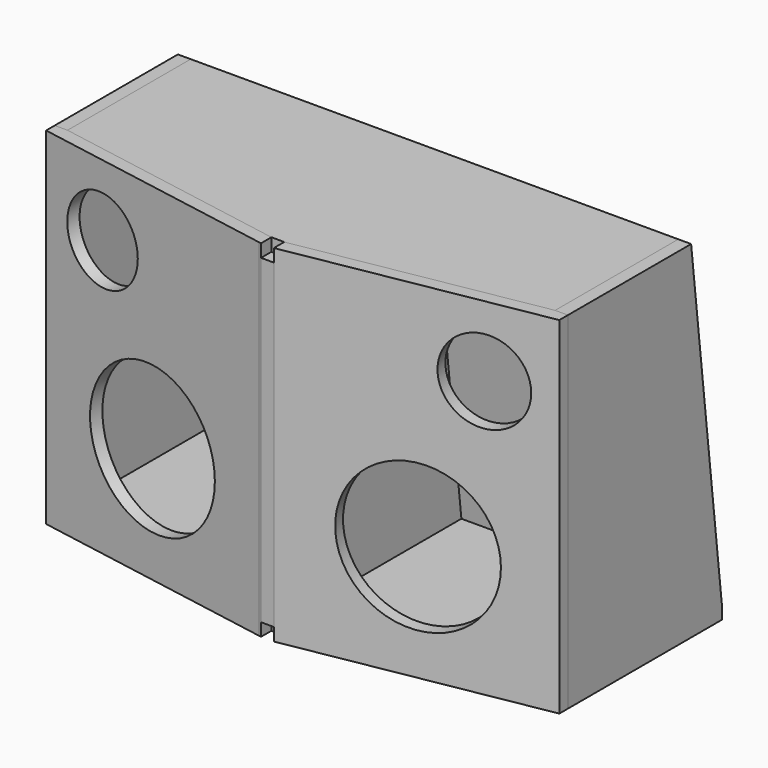
from build123d import *

# Parameters (mm, degrees)
F0_W      = 10
F0_H      = 120
F0_W_2    = 380
F0_H_2    = 10
F1_DEPTH  = 10
F2_DEPTH  = 270
F3_DEPTH  = 270
F6_W      = 150
F6_H      = 10
F7_DEPTH  = 10
F8_W      = 150
F8_H      = 10
F9_DEPTH  = 10
F11_DEPTH = 380
F12_DEPTH = 10
F13_R     = 32.5
F13_R_2   = 57.5
F14_DEPTH = 25
F15_R     = 57.5
F15_R_2   = 32.5
F16_DEPTH = 25
F17_W     = 10.1542661189
F17_H     = 250
F18_DEPTH = 10
F20_DEPTH = 380


# Not quite as in the source:
# - a feature names something its author has since deleted; it is built from what else it names


with BuildPart() as f1:
    # F0 (on Top) → F1 (new body)
    with BuildSketch(Plane.XY):
        Polygon((380, -10), (0, -10), (0, -150), (185, -182.6204914311), (185, -62.6204914311), (195, -62.6204914311), (195, -182.6204914311), (380, -150), align=None)
        with Locations((190, -122.6204914311)):
            Rectangle(F0_W, F0_H)
        with Locations((190, -5)):
            Rectangle(F0_W_2, F0_H_2)
    extrude(amount=F1_DEPTH)


with BuildPart() as f2:
    # F0 (on Top) → F2 (new body)
    with BuildSketch(Plane.XY):
        Polygon((185, -182.6204914311), (0, -150), (-10, -150), (-10, -158.3909963118), (183.2635182233, -192.4685689612), (185, -192.7747575499), align=None)
    extrude(amount=F2_DEPTH)

    # F13 (on face) → F14 (cut)
    with BuildSketch(Plane(origin=(-27.3879925261, -155.3250240891, 0), x_dir=(0.984807753, -0.1736481777, 0), z_dir=(-0.1736481777, -0.984807753, 0))):
        with Locations((69.6562303383, 215)):
            Circle(F13_R)
        with Locations((115.6562303383, 90)):
            Circle(F13_R_2)
    extrude(amount=-F14_DEPTH, mode=Mode.SUBTRACT)


with BuildPart() as f3:
    # F0 (on Top) → F3 (new body)
    with BuildSketch(Plane.XY):
        Polygon((390, -150), (380, -150), (195, -182.6204914311), (195, -192.7747575499), (390, -158.3909963118), align=None)
    extrude(amount=F3_DEPTH)

    # F15 (on face) → F16 (cut)
    with BuildSketch(Plane(origin=(38.8463945768, -220.3088513209, 0), x_dir=(0.984807753, 0.1736481777, 0), z_dir=(0.1736481777, -0.984807753, 0))):
        with Locations((258.5707158064, 90)):
            Circle(F15_R)
        with Locations((304.5707158064, 215)):
            Circle(F15_R_2)
    extrude(amount=-F16_DEPTH, mode=Mode.SUBTRACT)


with BuildPart() as f7:
    # F6 (on face) → F7 (new body)
    with BuildSketch(Plane(origin=(0, 0, 0), x_dir=(0, -1, 0), z_dir=(-1, 0, 0))):
        with Locations((75, 5)):
            Rectangle(F6_W, F6_H)
        Polygon((30, 270), (0, 10), (150, 10), (150, 270), align=None)
    extrude(amount=F7_DEPTH)


with BuildPart() as f9:
    # F8 (on face) → F9 (new body)
    with BuildSketch(Plane.YZ.offset(380)):
        with Locations((-75, 5)):
            Rectangle(F8_W, F8_H)
        Polygon((-150, 270), (-150, 10), (0, 10), (-30, 270), align=None)
    extrude(amount=F9_DEPTH)


with BuildPart() as f11:
    # F10 (on face) → F11 (new body)
    with BuildSketch(Plane.YZ):
        Polygon((0, 10), (-28.8461538462, 260), (-38.912501791, 260), (-10.0663479448, 10), align=None)
    extrude(amount=F11_DEPTH)


with BuildPart() as f12:
    # F5 (on offset) → F12 (new body)
    with BuildSketch(Plane.XY.offset(260)):
        Polygon((195, -182.6204914311), (380, -150), (380, -30), (0, -30), (0, -150), (185, -182.6204914311), align=None)
    extrude(amount=F12_DEPTH)

    # F19 (on face) → F20 (join)
    with BuildSketch(Plane(origin=(380, 0, 0), x_dir=(0, -1, 0), z_dir=(-1, 0, 0))):
        Polygon((30, 260), (30, 270), (28.8461538462, 260), align=None)
    extrude(amount=F20_DEPTH)


with BuildPart() as f18:
    # F17 (on face) → F18 (new body)
    with BuildSketch(Plane.YZ.offset(185)):
        with Locations((-187.6976244905, 135)):
            Rectangle(F17_W, F17_H)
        Polygon((-10.0663479448, 10), (-38.912501791, 260), (-182.6204914311, 260), (-182.6204914311, 10), (-150, 10), align=None)
    extrude(amount=F18_DEPTH)


solid = Compound([f1.part, f2.part, f3.part, f7.part, f9.part, f11.part, f12.part, f18.part])
